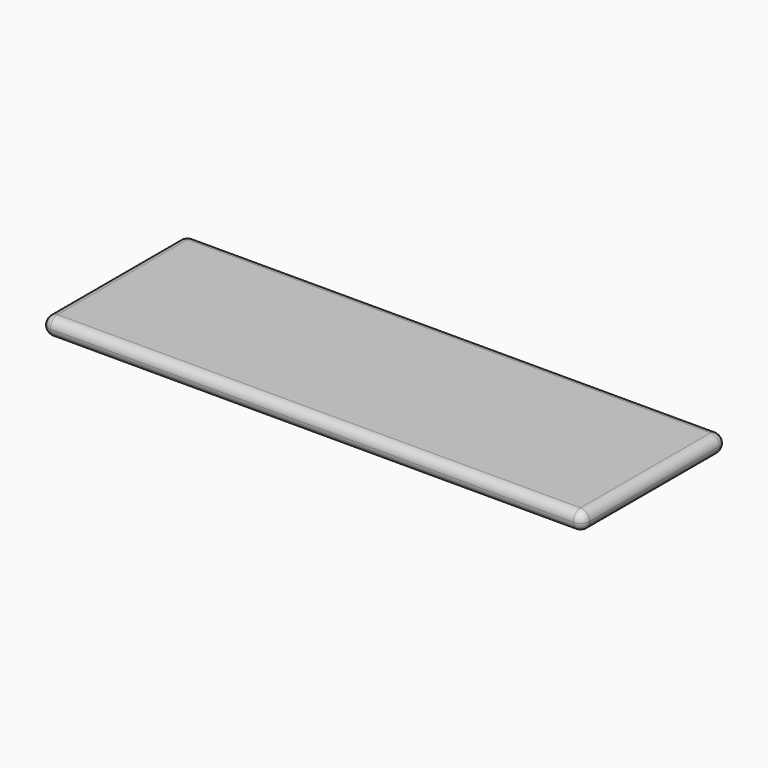
from build123d import *

# Parameters (mm, degrees)
F0_W     = 30
F0_H     = 10
F1_DEPTH = 1
F2_R     = 0.49999


# Not quite as in the source:
# - a fillet or chamfer is up to 0.001 mm smaller than in the source, because OpenCascade refuses the exact size


with BuildPart() as f1:
    # F0 (on Top) → F1 (new body)
    with BuildSketch(Plane.XY):
        with Locations((-34.182050813, 30.2290999105)):
            Rectangle(F0_W, F0_H)
    extrude(amount=F1_DEPTH)

    # F2 (radius 0.5 in the source; OpenCascade refuses exactly that, so slightly less here)
    f2_edges = [f1.edges().sort_by_distance(p)[0] for p in [
        (-34.182051, 35.2291, 1),
        (-49.182051, 30.2291, 1),
        (-34.182051, 25.2291, 1),
        (-19.182051, 30.2291, 1),
        (-19.182051, 35.2291, 0.5),
        (-34.182051, 35.2291, 0),
        (-49.182051, 35.2291, 0.5),
        (-49.182051, 30.2291, 0),
        (-49.182051, 25.2291, 0.5),
        (-34.182051, 25.2291, 0),
        (-19.182051, 25.2291, 0.5),
        (-19.182051, 30.2291, 0),
    ]]
    fillet(f2_edges, radius=F2_R)


solid = f1.part
